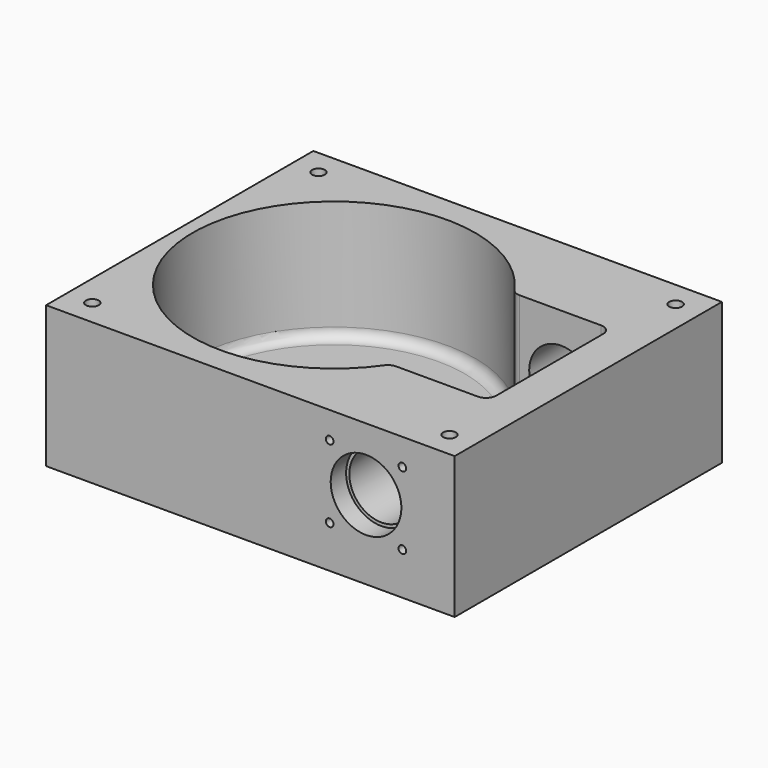
from build123d import *

# Parameters (mm, degrees)
F2_W      = 201.93
F2_H      = 70.01637
F3_DEPTH  = 82.55
F5_DEPTH  = 59.69762
F6_R      = 12.7
F7_DEPTH  = 6.35
F8_R      = 6.477
F9_DEPTH  = 25.4
F10_R     = 15.875
F11_DEPTH = 165.101
F12_R     = 3.175
F13_DEPTH = 70.01737
F15_R     = 1.89865
F16_DEPTH = 12.7
F14_R     = 17.4625
F17_DEPTH = 9.525
F18_R     = 5.08


# Not quite as in the source:
# - a pattern or mirror of a feature is missing from the dataset's text; its kind, count and spacing are read off the source's solid


with BuildPart() as f3:
    # F2 (on Front) → F3 (new body, symmetric)
    with BuildSketch(Plane.XZ):
        with Locations((24.765, -3.893185)):
            Rectangle(F2_W, F2_H)
    extrude(amount=F3_DEPTH, both=True)

    # F4 (on face) → F5 (cut)
    with BuildSketch(Plane.XY.offset(31.115)):
        with BuildLine():
            Line((106.68, 38.1), (58.5441073038, 38.1))
            ThreePointArc((58.5441073038, 38.1), (-69.85, 0), (58.5441073038, -38.1))
            Line((58.5441073038, -38.1), (106.68, -38.1))
            Line((106.68, -38.1), (106.68, 38.1))
        make_face()
    extrude(amount=-F5_DEPTH, mode=Mode.SUBTRACT)

    # F6 (on face) → F7 (cut)
    with BuildSketch(Plane(origin=(0, 0, -38.90137), x_dir=(1, 0, 0), z_dir=(0, 0, -1))):
        Circle(F6_R)
    extrude(amount=-F7_DEPTH, mode=Mode.SUBTRACT)

    # F8 (on face) → F9 (cut)
    with BuildSketch(Plane(origin=(0, 0, -32.55137), x_dir=(1, 0, 0), z_dir=(0, 0, -1))):
        Circle(F8_R)
    extrude(amount=-F9_DEPTH, mode=Mode.SUBTRACT)

    # F10 (on face) → F11 (cut, through all)
    with BuildSketch(Plane(origin=(0, 82.55, 0), x_dir=(-1, 0, 0), z_dir=(0, 1, 0))):
        with Locations((-81.915, 0)):
            Circle(F10_R)
    extrude(amount=-F11_DEPTH, mode=Mode.SUBTRACT)

    # F12 (on face) → F13 (cut, through all)
    with BuildSketch(Plane.XY.offset(31.115)):
        with Locations((-63.5, 69.85)):
            Circle(F12_R)
        with Locations((-63.5, -69.85)):
            Circle(F12_R)
        with Locations((113.03, 69.85)):
            Circle(F12_R)
        with Locations((113.03, -69.85)):
            Circle(F12_R)
    extrude(amount=-F13_DEPTH, mode=Mode.SUBTRACT)

    # F15 (on face) → F16 (cut)
    with BuildSketch(Plane(origin=(0, 82.55, 0), x_dir=(-1, 0, 0), z_dir=(0, 1, 0))):
        with Locations((-99.8755122421, 17.9605122421)):
            Circle(F15_R)
        with Locations((-99.8755122421, -17.9605122421)):
            Circle(F15_R)
        with Locations((-63.9544877579, -17.9605122421)):
            Circle(F15_R)
        with Locations((-63.9544877579, 17.9605122421)):
            Circle(F15_R)
    f16 = extrude(amount=-F16_DEPTH, mode=Mode.SUBTRACT)

    # F16_copies: F16 across plane
    add(f16.mirror(Plane(origin=(0, 0, 0), x_dir=(0, 0, -1), z_dir=(0, -1, 0))), mode=Mode.SUBTRACT)

    # F14 (on face) → F17 (cut)
    with BuildSketch(Plane(origin=(0, 82.55, 0), x_dir=(-1, 0, 0), z_dir=(0, 1, 0))):
        with Locations((-81.915, 0)):
            Circle(F14_R)
    f17 = extrude(amount=-F17_DEPTH, mode=Mode.SUBTRACT)

    # F17_copies: F17 across plane
    add(f17.mirror(Plane(origin=(0, 0, 0), x_dir=(0, 0, -1), z_dir=(0, -1, 0))), mode=Mode.SUBTRACT)

    # F18
    f18_edges = [f3.edges().sort_by_distance(p)[0] for p in [
        (-69.85, 0, -28.58262),
        (82.612054, 38.1, -28.58262),
        (106.68, 0, -28.58262),
        (82.612054, -38.1, -28.58262),
        (58.544107, 38.1, 1.26619),
        (58.544107, -38.1, 1.26619),
        (106.68, 38.1, 1.26619),
        (106.68, -38.1, 1.26619),
    ]]
    fillet(f18_edges, radius=F18_R)


solid = f3.part
